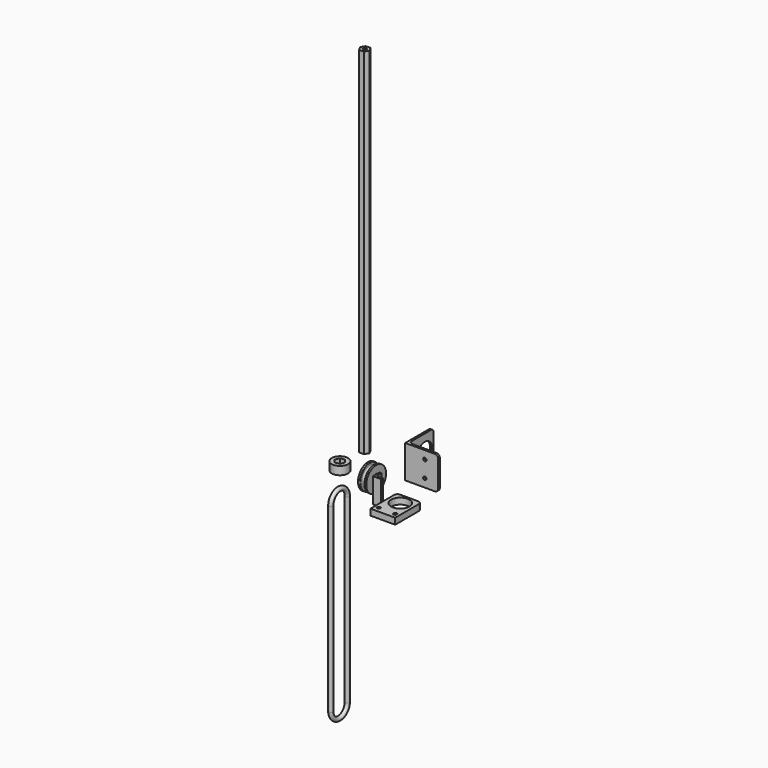
from build123d import *

# Parameters (mm, degrees)
F0_R      = 2.5527
F1_DEPTH  = 546.1
F5_DEPTH  = 69.0860653766
F6_R      = 0.635
F7_R      = 12.7
F8_DEPTH  = 12.7
F10_R     = 3.175
F13_DEPTH = 50.8
F15_R     = 2.5527
F16_DEPTH = 113.1975139048
F14_R     = 14.2875
F17_DEPTH = 95.533682572
F18_R     = 5.08
F20_DEPTH = 38.1
F21_R     = 2.5527
F22_DEPTH = 103.9870133122
F23_W     = 38.1
F23_H     = 50.8
F23_R     = 2.5527
F23_R_2   = 14.2875
F24_DEPTH = 9.525
F25_R     = 5.08


# Not quite as in the source:
# - a length typed as a fraction of an inch, garbled in the dataset ("3 / 203.2 mm" for 3/8 in), is restored


with BuildPart() as f1:
    # F0 (on Top) → F1 (new body)
    with BuildSketch(Plane.XY):
        Polygon((-59.5808195147, 49.0649654818), (-52.2485542758, 49.0300398551), (-48.5521751764, 55.3625050059), (-52.1880613159, 61.7298957835), (-59.5203265548, 61.7648214102), (-63.2167056542, 55.4323562593), align=None)
        with Locations((-55.8844404153, 55.3974306326)):
            Circle(F0_R, mode=Mode.SUBTRACT)
    extrude(amount=F1_DEPTH)


with BuildPart() as f3:
    # F2 (on Front) → F3 (revolve)
    with BuildSketch(Plane.XZ):
        with BuildLine():
            Line((-6.8316402776, 24.1360249974), (-6.8316402776, 5.0860249974))
            Line((-6.8316402776, 5.0860249974), (5.8683597224, 5.0860249974))
            Line((5.8683597224, 5.0860249974), (5.8683597224, 24.1360249974))
            Line((5.8683597224, 24.1360249974), (2.6933597224, 24.1360249974))
            Line((2.6933597224, 24.1360249974), (2.6933597224, 20.9610249974))
            ThreePointArc((2.6933597224, 20.9610249974), (-0.4816402776, 17.7860249974), (-3.6566402776, 20.9610249974))
            Line((-3.6566402776, 20.9610249974), (-3.6566402776, 24.1360249974))
            Line((-3.6566402776, 24.1360249974), (-6.8316402776, 24.1360249974))
        make_face()
    revolve(axis=Axis((-0.4816402776, 0, 5.0860249974), (-1, 0, 0)))

    # F4 (on face) → F5 (cut, through all)
    with BuildSketch(Plane.YZ.offset(5.8683597224)):
        Polygon((0, 12.4183734161), (-6.35, 8.7521992068), (-6.35, 1.4198507881), (0, -2.2463234213), (6.35, 1.4198507881), (6.35, 8.7521992068), align=None)
    extrude(amount=-F5_DEPTH, mode=Mode.SUBTRACT)

    # F6
    f6_edges = [f3.edges().sort_by_distance(p)[0] for p in [
        (-3.65664, 0, -13.963975),
        (2.69336, 0, -13.963975),
    ]]
    fillet(f6_edges, radius=F6_R)


with BuildPart() as f8:
    # F7 (on Top) → F8 (new body)
    with BuildSketch(Plane.XY):
        with Locations((-48.3974553645, -1.9041541964)):
            Circle(F7_R)
        Polygon((-43.8293768809, -7.6396569905), (-51.0805072459, -8.7279776067), (-55.6485857294, -2.9924748126), (-52.965533848, 3.8313485977), (-45.714403483, 4.9196692139), (-41.1463249995, -0.8158335802), align=None, mode=Mode.SUBTRACT)
    extrude(amount=F8_DEPTH)


with BuildPart() as f11:
    # F11: sweep along a path in F9
    with BuildLine(Plane.YZ) as f11_path:
        ThreePointArc((-79.9983394444, 0), (-64.1233394444, 15.875), (-48.2483394444, 0))
        Line((-48.2483394444, 0), (-48.2483394444, -279.4))
        ThreePointArc((-48.2483394444, -279.4), (-64.1233394444, -295.275), (-79.9983394444, -279.4))
        Line((-79.9983394444, -279.4), (-79.9983394444, 0))
    # F10 (on Top) → F11 (sweep)
    with BuildSketch(Plane.XY):
        with Locations((0, -79.9983394444)):
            Circle(F10_R)
    sweep(path=f11_path.line)


with BuildPart() as f13:
    # F12 (on Top) → F13 (new body)
    with BuildSketch(Plane.XY):
        with BuildLine():
            Line((32.3159769177, 77.6481743604), (29.1409769177, 77.6481743604))
            Line((29.1409769177, 77.6481743604), (29.1409769177, 26.8481743604))
            Line((29.1409769177, 26.8481743604), (79.9409769177, 26.8481743604))
            Line((79.9409769177, 26.8481743604), (79.9409769177, 30.0231743604))
            Line((79.9409769177, 30.0231743604), (38.6659769177, 30.0231743604))
            ThreePointArc((38.6659769177, 30.0231743604), (34.1758488572, 31.8830462999), (32.3159769177, 36.3731743604))
            Line((32.3159769177, 36.3731743604), (32.3159769177, 77.6481743604))
        make_face()
    extrude(amount=F13_DEPTH)

    # F15 (on face) → F16 (cut, through all)
    with BuildSketch(Plane(origin=(0, 30.0231743604, 0), x_dir=(-1, 0, 0), z_dir=(0, 1, 0))):
        with Locations((-59.3034769177, 38.1)):
            Circle(F15_R)
        with Locations((-59.3034769177, 12.7)):
            Circle(F15_R)
    extrude(amount=-F16_DEPTH, mode=Mode.SUBTRACT)

    # F14 (on face) → F17 (cut, through all)
    with BuildSketch(Plane.YZ.offset(32.3159769177)):
        with Locations((60.5031743604, 25.4)):
            Circle(F14_R)
    extrude(amount=-F17_DEPTH, mode=Mode.SUBTRACT)

    # F18
    f18_edges = [f13.edges().sort_by_distance(p)[0] for p in [
        (30.728477, 77.648174, 50.8),
        (30.728477, 77.648174, 0),
        (79.940977, 28.435674, 50.8),
        (79.940977, 28.435674, 0),
    ]]
    fillet(f18_edges, radius=F18_R)


with BuildPart() as f20:
    # F19 (on Top) → F20 (new body)
    with BuildSketch(Plane.XY):
        Polygon((40.7693076579, -33.2303968845), (37.5943076579, -33.2303968845), (37.5943076579, -45.9303968845), (50.2943076579, -45.9303968845), (50.2943076579, -42.7553968845), (40.7693076579, -42.7553968845), align=None)
    extrude(amount=F20_DEPTH)

    # F21 (on face) → F22 (cut, through all)
    with BuildSketch(Plane.YZ.offset(40.7693076579)):
        with Locations((-37.9928968845, 31.75)):
            Circle(F21_R)
        with Locations((-37.9928968845, 6.35)):
            Circle(F21_R)
    extrude(amount=-F22_DEPTH, mode=Mode.SUBTRACT)


with BuildPart() as f24:
    # F23 (on Top) → F24 (new body)
    with BuildSketch(Plane.XY):
        with Locations((72.8961580873, -45.5793716669)):
            Rectangle(F23_W, F23_H)
        with Locations((60.1961580873, -63.0418716669)):
            Circle(F23_R, mode=Mode.SUBTRACT)
        with Locations((85.5961580873, -63.0418716669)):
            Circle(F23_R, mode=Mode.SUBTRACT)
        with Locations((72.8961580873, -37.3243716669)):
            Circle(F23_R_2, mode=Mode.SUBTRACT)
    extrude(amount=F24_DEPTH)

    # F25
    f25_edges = [f24.edges().sort_by_distance(p)[0] for p in [
        (53.846158, -20.179372, 4.7625),
        (91.946158, -20.179372, 4.7625),
    ]]
    fillet(f25_edges, radius=F25_R)


solid = Compound([f1.part, f3.part, f8.part, f11.part, f13.part, f20.part, f24.part])
